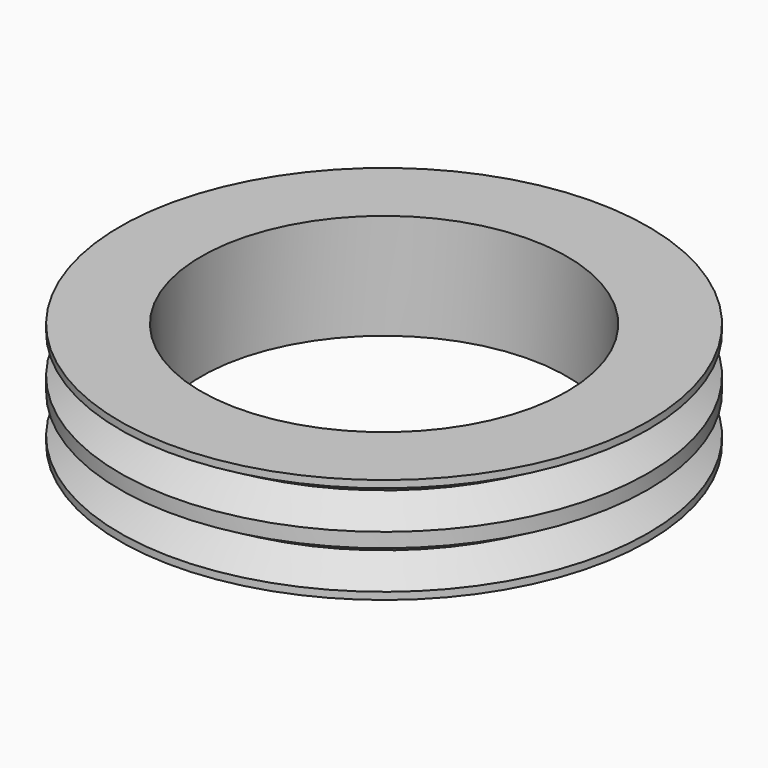
from build123d import *

# Parameters (mm, degrees)
F0_R     = 15.875
F0_R_2   = 11
F1_DEPTH = 6.35


# Not quite as in the source:
# - a length typed as a fraction of an inch, garbled in the dataset ("3 / 203.2 mm" for 3/8 in), is restored


with BuildPart() as f1:
    # F0 (on Top) → F1 (new body)
    with BuildSketch(Plane.XY):
        Circle(F0_R)
        Circle(F0_R_2, mode=Mode.SUBTRACT)
    extrude(amount=F1_DEPTH)

    # F2 (on Front) → F3 (revolve, cut)
    with BuildSketch(Plane.XZ):
        Polygon((15.875, 0.4327994616), (15.875, 2.7422005384), (13.875, 1.5875), align=None)
        Polygon((15.875, 5.9172005384), (13.875, 4.7625), (15.875, 3.6077994616), align=None)
    revolve(axis=Axis((0, 0, 9.5765832812), (0, 0, 1)), mode=Mode.SUBTRACT)


solid = f1.part
